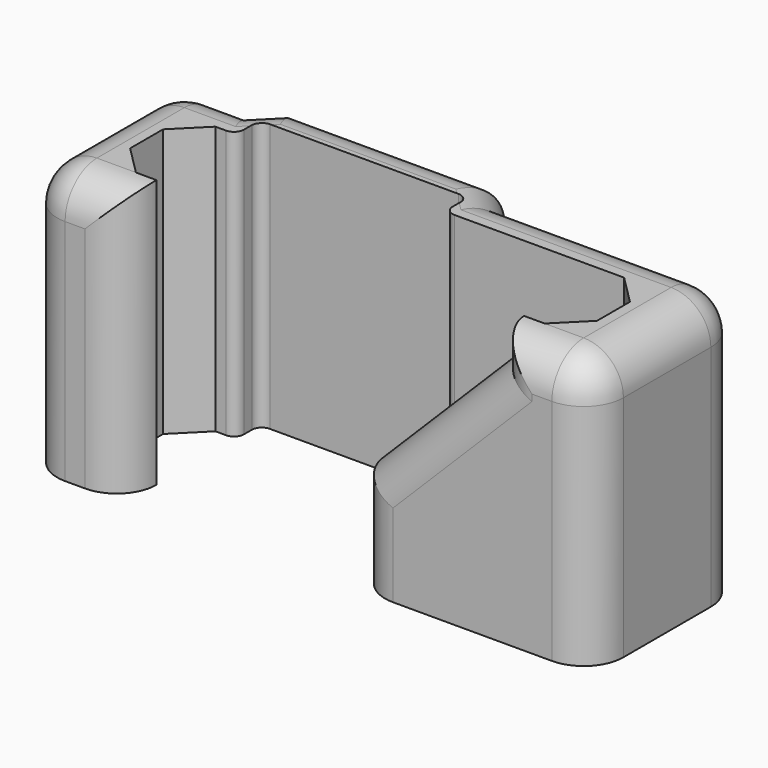
from build123d import *

# Parameters (mm, degrees)
F0_W           = 10
F0_H           = 17
F0_H_2         = 10
F0_W_2         = 23
F1_DEPTH       = 5
F2_DEPTH       = 14
F4_DEPTH       = 35
F8_DEPTH       = 27.001
F8_DEPTH_BACK  = 35
F10_W          = 27
F10_H          = 3
F11_DEPTH      = 21
F13_DEPTH      = 27
F14_R          = 1
F15_T1_DEPTH   = 11
F15_T3_DEPTH   = 6
F15_T5_DEPTH   = 23
F15_T7_DEPTH   = 6
F15_T9_DEPTH   = 27
F15_S13_W      = 4.08
F15_S13_H      = 4.08
F15_T14_DEPTH  = 4.08
F15_S19_W      = 4.08
F15_S19_H      = 4.08
F15_T20_DEPTH  = 4.08
F15_S25_W      = 4.08
F15_S25_H      = 4.08
F15_T26_DEPTH  = 4.08
F15_S31_W      = 4.08
F15_S31_H      = 4.08
F15_T32_DEPTH  = 4.08
F15_T38_DEPTH  = 13
F15_T43_DEPTH  = 39.7989898732
F15_T49_DEPTH  = 20
F15_T54_DEPTH  = 29.5
F15_T59_DEPTH  = 23.5355339059
F15_T65_DEPTH  = 41
F15_T71_DEPTH  = 23.5355339059
F15_T77_DEPTH  = 13.5
F15_T83_DEPTH  = 16
F15_T87_DEPTH  = 23
F15_T95_DEPTH  = 16
F15_T99_DEPTH  = 37
F15_T106_DEPTH = 13
F15_T110_DEPTH = 39.7989898732
F15_T117_DEPTH = 20
F15_T121_DEPTH = 39.7989898732
F15_T128_DEPTH = 29.5
F15_T132_DEPTH = 23.5355339059
F15_T139_DEPTH = 23.5355339059
F15_T143_DEPTH = 41
F15_T150_DEPTH = 41
F15_T154_DEPTH = 23.5355339059
F15_T161_DEPTH = 23.5355339059
F15_T165_DEPTH = 13.5
F16_ANGLE      = 270


# Not quite as in the source:
# - a fillet or chamfer that OpenCascade refuses, or shapes differently, is made with other operations: its cross-section is extruded or revolved along the edge and cut away or added


with BuildPart() as f1:
    # F0 (on Top) → F1 (new body)
    with BuildSketch(Plane.XY):
        Polygon((37, 0), (0, 0), (0, -17), (23, -17), (37, -3), align=None)
        with Locations((-5, -8.5)):
            Rectangle(F0_W, F0_H)
        Polygon((37, -17), (23, -17), (23, -27), (47, -27), (47, -17), align=None)
        with Locations((-5, -22)):
            Rectangle(F0_W, F0_H_2)
        Polygon((47, 0), (37, 0), (37, -3), (37, -17), (47, -17), align=None)
        with Locations((11.5, -22)):
            Rectangle(F0_W_2, F0_H_2)
        Polygon((37, -17), (37, -3), (23, -17), align=None)
    extrude(amount=-F1_DEPTH)

    # F0 (on Top) → F2 (join)
    with BuildSketch(Plane.XY):
        with Locations((-5, -8.5)):
            Rectangle(F0_W, F0_H)
        Polygon((47, 0), (37, 0), (37, -3), (37, -17), (47, -17), align=None)
        Polygon((37, -17), (37, -3), (23, -17), align=None)
        Polygon((37, -17), (23, -17), (23, -27), (47, -27), (47, -17), align=None)
        with Locations((-5, -22)):
            Rectangle(F0_W, F0_H_2)
    extrude(amount=F2_DEPTH)

    # F3 (on face) → F4 (cut)
    with BuildSketch(Plane(origin=(0, 0, 0), x_dir=(-1, 0, 0), z_dir=(0, 1, 0))):
        Polygon((2.0710678119, 0), (5, 2.9289321881), (5, 7.0710678119), (2.0710678119, 10), (0, 10), (0, 0), align=None)
    extrude(amount=-F4_DEPTH, mode=Mode.SUBTRACT)

    # F7: sweep along a path in F6
    with BuildLine(Plane.XY.offset(4.5)) as f7_path:
        Line((37, 0), (37, -3))
        Line((37, -3), (23, -17))
        Line((23, -17), (19.396028844, -20.603971156))
    # F3 (on face) → F7 (sweep, cut)
    with BuildSketch(Plane(origin=(0, 0, 0), x_dir=(-1, 0, 0), z_dir=(0, 1, 0))):
        with BuildLine():
            Line((-39.0710678119, 0), (-37, 0))
            Line((-37, 0), (-37, 1))
            ThreePointArc((-37, 1), (-41, 5), (-37, 9))
            Line((-37, 9), (-37, 10))
            Line((-37, 10), (-39.0710678119, 10))
            Line((-39.0710678119, 10), (-42, 7.0710678119))
            Line((-42, 7.0710678119), (-42, 2.9289321881))
            Line((-42, 2.9289321881), (-39.0710678119, 0))
        make_face()
        with BuildLine():
            ThreePointArc((-37, 9), (-41, 5), (-37, 1))
            Line((-37, 1), (-37, 9))
        make_face()
    sweep(path=f7_path.line, transition=Transition.RIGHT, mode=Mode.SUBTRACT)

    # F3 (on face) → F8 (cut, two sides)
    with BuildSketch(Plane(origin=(0, 0, 0), x_dir=(-1, 0, 0), z_dir=(0, 1, 0))) as f8_sk:
        with BuildLine():
            Line((-37, 9), (-37, 1))
            ThreePointArc((-37, 1), (-34.1715728753, 2.1715728753), (-33, 5))
            ThreePointArc((-33, 5), (-34.1715728753, 7.8284271247), (-37, 9))
        make_face()
        with BuildLine():
            ThreePointArc((-37, 9), (-41, 5), (-37, 1))
            Line((-37, 1), (-37, 9))
        make_face()
    extrude(amount=-F8_DEPTH, mode=Mode.SUBTRACT)
    extrude(f8_sk.sketch, amount=F8_DEPTH_BACK, mode=Mode.SUBTRACT)

    # F10 (on offset) → F11 (cut)
    with BuildSketch(Plane(origin=(0, 0, 0), x_dir=(0, -1, 0), z_dir=(-1, 0, 0))):
        with Locations((13.5, -1.5)):
            Rectangle(F10_W, F10_H)
    extrude(amount=-F11_DEPTH, mode=Mode.SUBTRACT)

    # F12 (on face) → F13 (join, through all)
    with BuildSketch(Plane.XZ.offset(27)):
        Polygon((21, -7.5), (23.5, -5), (-2.5, -5), (0, -7.5), align=None)
    extrude(amount=-F13_DEPTH)

    # F14
    f14_edges = [f1.edges().sort_by_distance(p)[0] for p in [
        (0, -13.5, 0),
        (21, -13.5, 0),
        (21, -13.5, -3),
        (0, -13.5, -3),
    ]]
    fillet(f14_edges, radius=F14_R)

    # F15: fillet of radius 4 on 17 edges, made by hand

    # F15_s2 → F15_t1 (cut)
    with BuildSketch(Plane.XY.offset(-1)):
        with BuildLine():
            ThreePointArc((-10, -4), (-8.8284271247, -1.1715728753), (-6, 0))
            Line((-6, 0), (-6, 0.08))
            Line((-6, 0.08), (-10.08, 0.08))
            Line((-10.08, 0.08), (-10.08, -4))
            Line((-10.08, -4), (-10, -4))
        make_face()
        with BuildLine():
            ThreePointArc((47, -4), (45.8284271247, -1.1715728753), (43, 0))
            Line((43, 0), (43, 0.08))
            Line((43, 0.08), (47.08, 0.08))
            Line((47.08, 0.08), (47.08, -4))
            Line((47.08, -4), (47, -4))
        make_face()
    extrude(amount=F15_T1_DEPTH, mode=Mode.SUBTRACT)

    # F15_s4 → F15_t3 (cut)
    with BuildSketch(Plane.YZ.offset(37)):
        with BuildLine():
            ThreePointArc((-4, 14), (-1.1715728753, 12.8284271247), (0, 10))
            Line((0, 10), (0.08, 10))
            Line((0.08, 10), (0.08, 14.08))
            Line((0.08, 14.08), (-4, 14.08))
            Line((-4, 14.08), (-4, 14))
        make_face()
    extrude(amount=F15_T3_DEPTH, mode=Mode.SUBTRACT)

    # F15_s6 → F15_t5 (cut)
    with BuildSketch(Plane.XZ.offset(4)):
        with BuildLine():
            ThreePointArc((43, 14), (45.8284271247, 12.8284271247), (47, 10))
            Line((47, 10), (47.08, 10))
            Line((47.08, 10), (47.08, 14.08))
            Line((47.08, 14.08), (43, 14.08))
            Line((43, 14.08), (43, 14))
        make_face()
        with BuildLine():
            ThreePointArc((47, -1), (45.8284271247, -3.8284271247), (43, -5))
            Line((43, -5), (43, -5.08))
            Line((43, -5.08), (47.08, -5.08))
            Line((47.08, -5.08), (47.08, -1))
            Line((47.08, -1), (47, -1))
        make_face()
        with BuildLine():
            ThreePointArc((-10, 10), (-8.8284271247, 12.8284271247), (-6, 14))
            Line((-6, 14), (-6, 14.08))
            Line((-6, 14.08), (-10.08, 14.08))
            Line((-10.08, 14.08), (-10.08, 10))
            Line((-10.08, 10), (-10, 10))
        make_face()
        with BuildLine():
            ThreePointArc((-6, -5), (-8.8284271247, -3.8284271247), (-10, -1))
            Line((-10, -1), (-10.08, -1))
            Line((-10.08, -1), (-10.08, -5.08))
            Line((-10.08, -5.08), (-6, -5.08))
            Line((-6, -5.08), (-6, -5))
        make_face()
    extrude(amount=F15_T5_DEPTH, mode=Mode.SUBTRACT)

    # F15_s8 → F15_t7 (cut)
    with BuildSketch(Plane.YZ.offset(-6)):
        with BuildLine():
            ThreePointArc((-4, 14), (-1.1715728753, 12.8284271247), (0, 10))
            Line((0, 10), (0.08, 10))
            Line((0.08, 10), (0.08, 14.08))
            Line((0.08, 14.08), (-4, 14.08))
            Line((-4, 14.08), (-4, 14))
        make_face()
    extrude(amount=F15_T7_DEPTH, mode=Mode.SUBTRACT)

    # F15_s10 → F15_t9 (cut)
    with BuildSketch(Plane.XZ):
        with BuildLine():
            ThreePointArc((-4, 14), (-1.1715728753, 12.8284271247), (0, 10))
            Line((0, 10), (0.08, 10))
            Line((0.08, 10), (0.08, 14.08))
            Line((0.08, 14.08), (-4, 14.08))
            Line((-4, 14.08), (-4, 14))
        make_face()
    extrude(amount=F15_T9_DEPTH, mode=Mode.SUBTRACT)


with BuildPart() as f15_tool12:
    # F15_s13 → F15_t14 (new body)
    with BuildSketch(Plane.XZ.offset(4)):
        with Locations((-8.04, 12.04)):
            Rectangle(F15_S13_W, F15_S13_H)
    extrude(amount=-F15_T14_DEPTH)

    # F15_s15 → F15_t16 (revolve, cut)
    with BuildSketch(Plane(origin=(-6, -4, 10), x_dir=(0.7071067812, 0, -0.7071067812), z_dir=(0.7071067812, 0, 0.7071067812))):
        with BuildLine():
            ThreePointArc((0, -4), (4, 0), (0, 4))
            Line((0, 4), (0, -4))
        make_face()
    revolve(axis=Axis((-6, -4, 10), (0, 1, 0)), mode=Mode.SUBTRACT)


with BuildPart() as f1_1:
    add(f1.part)

    # F15_t11: cut F15_tool12
    add(f15_tool12.part, mode=Mode.SUBTRACT)


with BuildPart() as f15_tool18:
    # F15_s19 → F15_t20 (new body)
    with BuildSketch(Plane.XY.offset(-1)):
        with Locations((-8.04, -1.96)):
            Rectangle(F15_S19_W, F15_S19_H)
    extrude(amount=-F15_T20_DEPTH)

    # F15_s21 → F15_t22 (revolve, cut)
    with BuildSketch(Plane(origin=(-6, -4, -1), x_dir=(0.7071067812, -0.7071067812, 0), z_dir=(0.7071067812, 0.7071067812, 0))):
        with BuildLine():
            ThreePointArc((0, -4), (4, 0), (0, 4))
            Line((0, 4), (0, -4))
        make_face()
    revolve(axis=Axis((-6, -4, -1), (0, 0, -1)), mode=Mode.SUBTRACT)


with BuildPart() as f1_2:
    add(f1_1.part)

    # F15_t17: cut F15_tool18
    add(f15_tool18.part, mode=Mode.SUBTRACT)


with BuildPart() as f15_tool24:
    # F15_s25 → F15_t26 (new body)
    with BuildSketch(Plane.XY.offset(-1)):
        with Locations((45.04, -1.96)):
            Rectangle(F15_S25_W, F15_S25_H)
    extrude(amount=-F15_T26_DEPTH)

    # F15_s27 → F15_t28 (revolve, cut)
    with BuildSketch(Plane(origin=(43, -4, -1), x_dir=(-0.7071067812, -0.7071067812, 0), z_dir=(0.7071067812, -0.7071067812, 0))):
        with BuildLine():
            ThreePointArc((0, -4), (4, 0), (0, 4))
            Line((0, 4), (0, -4))
        make_face()
    revolve(axis=Axis((43, -4, -1), (0, 0, -1)), mode=Mode.SUBTRACT)


with BuildPart() as f1_3:
    add(f1_2.part)

    # F15_t23: cut F15_tool24
    add(f15_tool24.part, mode=Mode.SUBTRACT)


with BuildPart() as f15_tool30:
    # F15_s31 → F15_t32 (new body)
    with BuildSketch(Plane.XZ.offset(4)):
        with Locations((45.04, 12.04)):
            Rectangle(F15_S31_W, F15_S31_H)
    extrude(amount=-F15_T32_DEPTH)

    # F15_s33 → F15_t34 (revolve, cut)
    with BuildSketch(Plane(origin=(43, -4, 10), x_dir=(-0.7071067812, 0, -0.7071067812), z_dir=(0.7071067812, 0, -0.7071067812))):
        with BuildLine():
            ThreePointArc((0, -4), (4, 0), (0, 4))
            Line((0, 4), (0, -4))
        make_face()
    revolve(axis=Axis((43, -4, 10), (0, 1, 0)), mode=Mode.SUBTRACT)


with BuildPart() as f1_4:
    add(f1_3.part)

    # F15_t29: cut F15_tool30
    add(f15_tool30.part, mode=Mode.SUBTRACT)


with BuildPart() as f15_tool36:
    # F15_s37 → F15_t38 (new body)
    with BuildSketch(Plane.XZ):
        with BuildLine():
            ThreePointArc((41, 14), (38.1715728753, 12.8284271247), (37, 10))
            Line((37, 10), (36.92, 10))
            Line((36.92, 10), (36.92, 14.08))
            Line((36.92, 14.08), (41, 14.08))
            Line((41, 14.08), (41, 14))
        make_face()
    extrude(amount=F15_T38_DEPTH)

    split(bisect_by=Plane(origin=(20, -20, 0), x_dir=(0, 0, 1), z_dir=(-0.7071067812, 0.7071067812, 0)), keep=Keep.TOP)


with BuildPart() as f1_5:
    add(f1_4.part)

    # F15_t35: cut F15_tool36
    add(f15_tool36.part, mode=Mode.SUBTRACT)


with BuildPart() as f15_tool41:
    # F15_s42 → F15_t43 (new body)
    with BuildSketch(Plane(origin=(24.0710678119, 24.0710678119, 0), x_dir=(0, 0, 1), z_dir=(-0.7071067812, -0.7071067812, 0))):
        with BuildLine():
            ThreePointArc((14, -32.2842712475), (12.8284271247, -29.4558441227), (10, -28.2842712475))
            Line((10, -28.2842712475), (10, -28.2042712475))
            Line((10, -28.2042712475), (14.08, -28.2042712475))
            Line((14.08, -28.2042712475), (14.08, -32.2842712475))
            Line((14.08, -32.2842712475), (14, -32.2842712475))
        make_face()
    extrude(amount=F15_T43_DEPTH)

    split(bisect_by=Plane.YZ.offset(23), keep=Keep.TOP)

    split(bisect_by=Plane.YZ.offset(37), keep=Keep.BOTTOM)


with BuildPart() as f1_6:
    add(f1_5.part)

    # F15_t40: cut F15_tool41
    add(f15_tool41.part, mode=Mode.SUBTRACT)


with BuildPart() as f15_tool47:
    # F15_s48 → F15_t49 (new body)
    with BuildSketch(Plane.XZ.offset(7)):
        with BuildLine():
            ThreePointArc((23, 10), (24.1715728753, 12.8284271247), (27, 14))
            Line((27, 14), (27, 14.08))
            Line((27, 14.08), (22.92, 14.08))
            Line((22.92, 14.08), (22.92, 10))
            Line((22.92, 10), (23, 10))
        make_face()
    extrude(amount=F15_T49_DEPTH)

    split(bisect_by=Plane(origin=(20, -20, 0), x_dir=(0, 0, 1), z_dir=(0.7071067812, -0.7071067812, 0)), keep=Keep.TOP)


with BuildPart() as f1_7:
    add(f1_6.part)

    # F15_t46: cut F15_tool47
    add(f15_tool47.part, mode=Mode.SUBTRACT)


with BuildPart() as f15_tool52:
    # F15_s53 → F15_t54 (new body)
    with BuildSketch(Plane.YZ.offset(43)):
        with BuildLine():
            ThreePointArc((-4, -5), (-1.1715728753, -3.8284271247), (0, -1))
            Line((0, -1), (0.08, -1))
            Line((0.08, -1), (0.08, -5.08))
            Line((0.08, -5.08), (-4, -5.08))
            Line((-4, -5.08), (-4, -5))
        make_face()
    extrude(amount=-F15_T54_DEPTH)

    split(bisect_by=Plane(origin=(14.25, 0, -14.25), x_dir=(0, 1, 0), z_dir=(0.7071067812, 0, -0.7071067812)), keep=Keep.TOP)


with BuildPart() as f1_8:
    add(f1_7.part)

    # F15_t51: cut F15_tool52
    add(f15_tool52.part, mode=Mode.SUBTRACT)


with BuildPart() as f15_tool57:
    # F15_s58 → F15_t59 (new body)
    with BuildSketch(Plane(origin=(-0.3210678119, 0, -0.3210678119), x_dir=(0, 1, 0), z_dir=(0.7071067812, 0, 0.7071067812))):
        with BuildLine():
            ThreePointArc((-4, -20.1525432638), (-1.1715728753, -18.9809703886), (0, -16.1525432638))
            Line((0, -16.1525432638), (0.08, -16.1525432638))
            Line((0.08, -16.1525432638), (0.08, -20.2325432638))
            Line((0.08, -20.2325432638), (-4, -20.2325432638))
            Line((-4, -20.2325432638), (-4, -20.1525432638))
        make_face()
    extrude(amount=F15_T59_DEPTH)

    split(bisect_by=Plane.XY.offset(-5), keep=Keep.BOTTOM)

    split(bisect_by=Plane.XY.offset(-7.5), keep=Keep.TOP)


with BuildPart() as f1_9:
    add(f1_8.part)

    # F15_t56: cut F15_tool57
    add(f15_tool57.part, mode=Mode.SUBTRACT)


with BuildPart() as f15_tool63:
    # F15_s64 → F15_t65 (new body)
    with BuildSketch(Plane.YZ.offset(-10)):
        with BuildLine():
            ThreePointArc((-4, -7.5), (-1.1715728753, -6.3284271247), (0, -3.5))
            Line((0, -3.5), (0.08, -3.5))
            Line((0.08, -3.5), (0.08, -7.58))
            Line((0.08, -7.58), (-4, -7.58))
            Line((-4, -7.58), (-4, -7.5))
        make_face()
    extrude(amount=F15_T65_DEPTH)

    split(bisect_by=Plane(origin=(14.25, 0, -14.25), x_dir=(0, 1, 0), z_dir=(-0.7071067812, 0, 0.7071067812)), keep=Keep.TOP)

    split(bisect_by=Plane(origin=(-3.75, 0, -3.75), x_dir=(0, 1, 0), z_dir=(0.7071067812, 0, 0.7071067812)), keep=Keep.TOP)


with BuildPart() as f1_10:
    add(f1_9.part)

    # F15_t62: cut F15_tool63
    add(f15_tool63.part, mode=Mode.SUBTRACT)


with BuildPart() as f15_tool69:
    # F15_s70 → F15_t71 (new body)
    with BuildSketch(Plane(origin=(-5.8210678119, 0, 5.8210678119), x_dir=(0, 1, 0), z_dir=(0.7071067812, 0, -0.7071067812))):
        with BuildLine():
            ThreePointArc((-4, -5.3033008589), (-1.1715728753, -4.1317279836), (0, -1.3033008589))
            Line((0, -1.3033008589), (0.08, -1.3033008589))
            Line((0.08, -1.3033008589), (0.08, -5.3833008589))
            Line((0.08, -5.3833008589), (-4, -5.3833008589))
            Line((-4, -5.3833008589), (-4, -5.3033008589))
        make_face()
    extrude(amount=F15_T71_DEPTH)

    split(bisect_by=Plane.XY.offset(-7.5), keep=Keep.TOP)

    split(bisect_by=Plane.XY.offset(-5), keep=Keep.BOTTOM)


with BuildPart() as f1_11:
    add(f1_10.part)

    # F15_t68: cut F15_tool69
    add(f15_tool69.part, mode=Mode.SUBTRACT)


with BuildPart() as f15_tool75:
    # F15_s76 → F15_t77 (new body)
    with BuildSketch(Plane.YZ.offset(7.5)):
        with BuildLine():
            ThreePointArc((-4, -5), (-1.1715728753, -3.8284271247), (0, -1))
            Line((0, -1), (0.08, -1))
            Line((0.08, -1), (0.08, -5.08))
            Line((0.08, -5.08), (-4, -5.08))
            Line((-4, -5.08), (-4, -5))
        make_face()
    extrude(amount=-F15_T77_DEPTH)

    split(bisect_by=Plane(origin=(-3.75, 0, -3.75), x_dir=(0, 1, 0), z_dir=(-0.7071067812, 0, -0.7071067812)), keep=Keep.TOP)


with BuildPart() as f1_12:
    add(f1_11.part)

    # F15_t74: cut F15_tool75
    add(f15_tool75.part, mode=Mode.SUBTRACT)


with BuildPart() as f15_tool81:
    # F15_s82 → F15_t83 (new body)
    with BuildSketch(Plane.YZ.offset(43)):
        with BuildLine():
            ThreePointArc((-4, 14), (-1.1715728753, 12.8284271247), (0, 10))
            Line((0, 10), (0.08, 10))
            Line((0.08, 10), (0.08, 14.08))
            Line((0.08, 14.08), (-4, 14.08))
            Line((-4, 14.08), (-4, 14))
        make_face()
    extrude(amount=-F15_T83_DEPTH)

    split(bisect_by=Plane.YZ.offset(37), keep=Keep.BOTTOM)


with BuildPart() as f15_tool85:
    # F15_s86 → F15_t87 (new body)
    with BuildSketch(Plane.XZ.offset(-10)):
        with BuildLine():
            ThreePointArc((41, 14), (38.1715728753, 12.8284271247), (37, 10))
            Line((37, 10), (36.92, 10))
            Line((36.92, 10), (36.92, 14.08))
            Line((36.92, 14.08), (41, 14.08))
            Line((41, 14.08), (41, 14))
        make_face()
    extrude(amount=F15_T87_DEPTH)

    split(bisect_by=Plane.XZ, keep=Keep.BOTTOM)

    split(bisect_by=Plane(origin=(20, -20, 0), x_dir=(0, 0, 1), z_dir=(-0.7071067812, 0.7071067812, 0)), keep=Keep.TOP)


with BuildPart() as f15_tool81_1:
    add(f15_tool81.part)

    # F15_t90: intersect F15_tool85
    add(f15_tool85.part, mode=Mode.INTERSECT)


with BuildPart() as f1_13:
    add(f1_12.part)

    # F15_t79: cut F15_tool81
    add(f15_tool81_1.part, mode=Mode.SUBTRACT)


with BuildPart() as f15_tool93:
    # F15_s94 → F15_t95 (new body)
    with BuildSketch(Plane.YZ.offset(10)):
        with BuildLine():
            ThreePointArc((-4, 14), (-1.1715728753, 12.8284271247), (0, 10))
            Line((0, 10), (0.08, 10))
            Line((0.08, 10), (0.08, 14.08))
            Line((0.08, 14.08), (-4, 14.08))
            Line((-4, 14.08), (-4, 14))
        make_face()
    extrude(amount=-F15_T95_DEPTH)

    split(bisect_by=Plane.YZ, keep=Keep.TOP)


with BuildPart() as f15_tool97:
    # F15_s98 → F15_t99 (new body)
    with BuildSketch(Plane.XZ.offset(27)):
        with BuildLine():
            ThreePointArc((-4, 14), (-1.1715728753, 12.8284271247), (0, 10))
            Line((0, 10), (0.08, 10))
            Line((0.08, 10), (0.08, 14.08))
            Line((0.08, 14.08), (-4, 14.08))
            Line((-4, 14.08), (-4, 14))
        make_face()
    extrude(amount=-F15_T99_DEPTH)

    split(bisect_by=Plane.XZ, keep=Keep.BOTTOM)


with BuildPart() as f15_tool93_1:
    add(f15_tool93.part)

    # F15_t101: intersect F15_tool97
    add(f15_tool97.part, mode=Mode.INTERSECT)


with BuildPart() as f1_14:
    add(f1_13.part)

    # F15_t91: cut F15_tool93
    add(f15_tool93_1.part, mode=Mode.SUBTRACT)


with BuildPart() as f15_tool104:
    # F15_s105 → F15_t106 (new body)
    with BuildSketch(Plane.XZ):
        with BuildLine():
            ThreePointArc((41, 14), (38.1715728753, 12.8284271247), (37, 10))
            Line((37, 10), (36.92, 10))
            Line((36.92, 10), (36.92, 14.08))
            Line((36.92, 14.08), (41, 14.08))
            Line((41, 14.08), (41, 14))
        make_face()
    extrude(amount=F15_T106_DEPTH)

    split(bisect_by=Plane(origin=(20, -20, 0), x_dir=(0, 0, 1), z_dir=(0.7071067812, -0.7071067812, 0)), keep=Keep.TOP)


with BuildPart() as f15_tool108:
    # F15_s109 → F15_t110 (new body)
    with BuildSketch(Plane(origin=(24.0710678119, 24.0710678119, 0), x_dir=(0, 0, 1), z_dir=(-0.7071067812, -0.7071067812, 0))):
        with BuildLine():
            ThreePointArc((14, -32.2842712475), (12.8284271247, -29.4558441227), (10, -28.2842712475))
            Line((10, -28.2842712475), (10, -28.2042712475))
            Line((10, -28.2042712475), (14.08, -28.2042712475))
            Line((14.08, -28.2042712475), (14.08, -32.2842712475))
            Line((14.08, -32.2842712475), (14, -32.2842712475))
        make_face()
    extrude(amount=F15_T110_DEPTH)

    split(bisect_by=Plane.YZ.offset(37), keep=Keep.TOP)


with BuildPart() as f15_tool104_1:
    add(f15_tool104.part)

    # F15_t112: intersect F15_tool108
    add(f15_tool108.part, mode=Mode.INTERSECT)


with BuildPart() as f1_15:
    add(f1_14.part)

    # F15_t102: cut F15_tool104
    add(f15_tool104_1.part, mode=Mode.SUBTRACT)


with BuildPart() as f15_tool115:
    # F15_s116 → F15_t117 (new body)
    with BuildSketch(Plane.XZ.offset(7)):
        with BuildLine():
            ThreePointArc((23, 10), (24.1715728753, 12.8284271247), (27, 14))
            Line((27, 14), (27, 14.08))
            Line((27, 14.08), (22.92, 14.08))
            Line((22.92, 14.08), (22.92, 10))
            Line((22.92, 10), (23, 10))
        make_face()
    extrude(amount=F15_T117_DEPTH)

    split(bisect_by=Plane(origin=(20, -20, 0), x_dir=(0, 0, 1), z_dir=(-0.7071067812, 0.7071067812, 0)), keep=Keep.TOP)


with BuildPart() as f15_tool119:
    # F15_s120 → F15_t121 (new body)
    with BuildSketch(Plane(origin=(24.0710678119, 24.0710678119, 0), x_dir=(0, 0, 1), z_dir=(-0.7071067812, -0.7071067812, 0))):
        with BuildLine():
            ThreePointArc((14, -32.2842712475), (12.8284271247, -29.4558441227), (10, -28.2842712475))
            Line((10, -28.2842712475), (10, -28.2042712475))
            Line((10, -28.2042712475), (14.08, -28.2042712475))
            Line((14.08, -28.2042712475), (14.08, -32.2842712475))
            Line((14.08, -32.2842712475), (14, -32.2842712475))
        make_face()
    extrude(amount=F15_T121_DEPTH)

    split(bisect_by=Plane.YZ.offset(23), keep=Keep.BOTTOM)


with BuildPart() as f15_tool115_1:
    add(f15_tool115.part)

    # F15_t123: intersect F15_tool119
    add(f15_tool119.part, mode=Mode.INTERSECT)


with BuildPart() as f1_16:
    add(f1_15.part)

    # F15_t113: cut F15_tool115
    add(f15_tool115_1.part, mode=Mode.SUBTRACT)


with BuildPart() as f15_tool126:
    # F15_s127 → F15_t128 (new body)
    with BuildSketch(Plane.YZ.offset(43)):
        with BuildLine():
            ThreePointArc((-4, -5), (-1.1715728753, -3.8284271247), (0, -1))
            Line((0, -1), (0.08, -1))
            Line((0.08, -1), (0.08, -5.08))
            Line((0.08, -5.08), (-4, -5.08))
            Line((-4, -5.08), (-4, -5))
        make_face()
    extrude(amount=-F15_T128_DEPTH)

    split(bisect_by=Plane(origin=(14.25, 0, -14.25), x_dir=(0, 1, 0), z_dir=(-0.7071067812, 0, 0.7071067812)), keep=Keep.TOP)


with BuildPart() as f15_tool130:
    # F15_s131 → F15_t132 (new body)
    with BuildSketch(Plane(origin=(-0.3210678119, 0, -0.3210678119), x_dir=(0, 1, 0), z_dir=(0.7071067812, 0, 0.7071067812))):
        with BuildLine():
            ThreePointArc((-4, -20.1525432638), (-1.1715728753, -18.9809703886), (0, -16.1525432638))
            Line((0, -16.1525432638), (0.08, -16.1525432638))
            Line((0.08, -16.1525432638), (0.08, -20.2325432638))
            Line((0.08, -20.2325432638), (-4, -20.2325432638))
            Line((-4, -20.2325432638), (-4, -20.1525432638))
        make_face()
    extrude(amount=F15_T132_DEPTH)

    split(bisect_by=Plane.XY.offset(-5), keep=Keep.TOP)


with BuildPart() as f15_tool126_1:
    add(f15_tool126.part)

    # F15_t134: intersect F15_tool130
    add(f15_tool130.part, mode=Mode.INTERSECT)


with BuildPart() as f1_17:
    add(f1_16.part)

    # F15_t124: cut F15_tool126
    add(f15_tool126_1.part, mode=Mode.SUBTRACT)


with BuildPart() as f15_tool137:
    # F15_s138 → F15_t139 (new body)
    with BuildSketch(Plane(origin=(-0.3210678119, 0, -0.3210678119), x_dir=(0, 1, 0), z_dir=(0.7071067812, 0, 0.7071067812))):
        with BuildLine():
            ThreePointArc((-4, -20.1525432638), (-1.1715728753, -18.9809703886), (0, -16.1525432638))
            Line((0, -16.1525432638), (0.08, -16.1525432638))
            Line((0.08, -16.1525432638), (0.08, -20.2325432638))
            Line((0.08, -20.2325432638), (-4, -20.2325432638))
            Line((-4, -20.2325432638), (-4, -20.1525432638))
        make_face()
    extrude(amount=F15_T139_DEPTH)

    split(bisect_by=Plane.XY.offset(-7.5), keep=Keep.BOTTOM)


with BuildPart() as f15_tool141:
    # F15_s142 → F15_t143 (new body)
    with BuildSketch(Plane.YZ.offset(-10)):
        with BuildLine():
            ThreePointArc((-4, -7.5), (-1.1715728753, -6.3284271247), (0, -3.5))
            Line((0, -3.5), (0.08, -3.5))
            Line((0.08, -3.5), (0.08, -7.58))
            Line((0.08, -7.58), (-4, -7.58))
            Line((-4, -7.58), (-4, -7.5))
        make_face()
    extrude(amount=F15_T143_DEPTH)

    split(bisect_by=Plane(origin=(14.25, 0, -14.25), x_dir=(0, 1, 0), z_dir=(0.7071067812, 0, -0.7071067812)), keep=Keep.TOP)


with BuildPart() as f15_tool137_1:
    add(f15_tool137.part)

    # F15_t145: intersect F15_tool141
    add(f15_tool141.part, mode=Mode.INTERSECT)


with BuildPart() as f1_18:
    add(f1_17.part)

    # F15_t135: cut F15_tool137
    add(f15_tool137_1.part, mode=Mode.SUBTRACT)


with BuildPart() as f15_tool148:
    # F15_s149 → F15_t150 (new body)
    with BuildSketch(Plane.YZ.offset(-10)):
        with BuildLine():
            ThreePointArc((-4, -7.5), (-1.1715728753, -6.3284271247), (0, -3.5))
            Line((0, -3.5), (0.08, -3.5))
            Line((0.08, -3.5), (0.08, -7.58))
            Line((0.08, -7.58), (-4, -7.58))
            Line((-4, -7.58), (-4, -7.5))
        make_face()
    extrude(amount=F15_T150_DEPTH)

    split(bisect_by=Plane(origin=(-3.75, 0, -3.75), x_dir=(0, 1, 0), z_dir=(-0.7071067812, 0, -0.7071067812)), keep=Keep.TOP)


with BuildPart() as f15_tool152:
    # F15_s153 → F15_t154 (new body)
    with BuildSketch(Plane(origin=(-5.8210678119, 0, 5.8210678119), x_dir=(0, 1, 0), z_dir=(0.7071067812, 0, -0.7071067812))):
        with BuildLine():
            ThreePointArc((-4, -5.3033008589), (-1.1715728753, -4.1317279836), (0, -1.3033008589))
            Line((0, -1.3033008589), (0.08, -1.3033008589))
            Line((0.08, -1.3033008589), (0.08, -5.3833008589))
            Line((0.08, -5.3833008589), (-4, -5.3833008589))
            Line((-4, -5.3833008589), (-4, -5.3033008589))
        make_face()
    extrude(amount=F15_T154_DEPTH)

    split(bisect_by=Plane.XY.offset(-7.5), keep=Keep.BOTTOM)


with BuildPart() as f15_tool148_1:
    add(f15_tool148.part)

    # F15_t156: intersect F15_tool152
    add(f15_tool152.part, mode=Mode.INTERSECT)


with BuildPart() as f1_19:
    add(f1_18.part)

    # F15_t146: cut F15_tool148
    add(f15_tool148_1.part, mode=Mode.SUBTRACT)


with BuildPart() as f15_tool159:
    # F15_s160 → F15_t161 (new body)
    with BuildSketch(Plane(origin=(-5.8210678119, 0, 5.8210678119), x_dir=(0, 1, 0), z_dir=(0.7071067812, 0, -0.7071067812))):
        with BuildLine():
            ThreePointArc((-4, -5.3033008589), (-1.1715728753, -4.1317279836), (0, -1.3033008589))
            Line((0, -1.3033008589), (0.08, -1.3033008589))
            Line((0.08, -1.3033008589), (0.08, -5.3833008589))
            Line((0.08, -5.3833008589), (-4, -5.3833008589))
            Line((-4, -5.3833008589), (-4, -5.3033008589))
        make_face()
    extrude(amount=F15_T161_DEPTH)

    split(bisect_by=Plane.XY.offset(-5), keep=Keep.TOP)


with BuildPart() as f15_tool163:
    # F15_s164 → F15_t165 (new body)
    with BuildSketch(Plane.YZ.offset(7.5)):
        with BuildLine():
            ThreePointArc((-4, -5), (-1.1715728753, -3.8284271247), (0, -1))
            Line((0, -1), (0.08, -1))
            Line((0.08, -1), (0.08, -5.08))
            Line((0.08, -5.08), (-4, -5.08))
            Line((-4, -5.08), (-4, -5))
        make_face()
    extrude(amount=-F15_T165_DEPTH)

    split(bisect_by=Plane(origin=(-3.75, 0, -3.75), x_dir=(0, 1, 0), z_dir=(0.7071067812, 0, 0.7071067812)), keep=Keep.TOP)


with BuildPart() as f15_tool159_1:
    add(f15_tool159.part)

    # F15_t167: intersect F15_tool163
    add(f15_tool163.part, mode=Mode.INTERSECT)


with BuildPart() as f1_20:
    add(f1_19.part)

    # F15_t157: cut F15_tool159
    add(f15_tool159_1.part, mode=Mode.SUBTRACT)


with BuildPart() as f1_21:
    # F16: moved
    add(f1_20.part.rotate(Axis((10.5, -27, -7.5), (-1, 0, 0)), F16_ANGLE))


solid = f1_21.part
